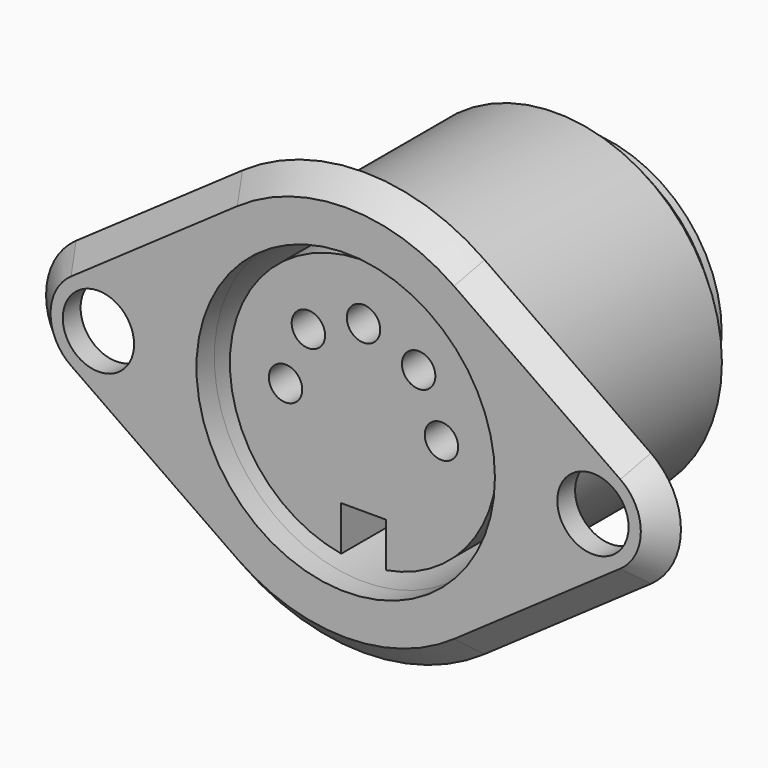
from build123d import *

# Parameters (mm, degrees)
F0_R     = 1.6
F0_R_2   = 7.45
F0_R_3   = 6.7
F1_DEPTH = 1
F2_SIZE  = 0.99999
F0_R_4   = 0.75
F3_DEPTH = 12.1
F4_T     = 0.75
F5_DEPTH = 12.6
F6_DEPTH = 10
F7_SIZE  = 1.3


# Not quite as in the source:
# - a fillet or chamfer is up to 0.001 mm smaller than in the source, because OpenCascade refuses the exact size
# - a shell that OpenCascade refuses in one call is made with other operations: the cavity is built on its own and cut out


with BuildPart() as f1:
    # F0 (on Front) → F1 (new body)
    with BuildSketch(Plane.XZ):
        with BuildLine():
            Line((-5.4346846847, 7.7919318771), (-12.902027027, 2.5836405698))
            ThreePointArc((-12.902027027, 2.5836405698), (-14.25, 0), (-12.902027027, -2.5836405698))
            Line((-12.902027027, -2.5836405698), (-5.4346846847, -7.7919318771))
            ThreePointArc((-5.4346846847, -7.7919318771), (0, -9.5), (5.4346846847, -7.7919318771))
            Line((5.4346846847, -7.7919318771), (12.902027027, -2.5836405698))
            ThreePointArc((12.902027027, -2.5836405698), (14.25, 0), (12.902027027, 2.5836405698))
            Line((12.902027027, 2.5836405698), (5.4346846847, 7.7919318771))
            ThreePointArc((5.4346846847, 7.7919318771), (0, 9.5), (-5.4346846847, 7.7919318771))
        make_face()
        with Locations((-11.1, 0)):
            Circle(F0_R, mode=Mode.SUBTRACT)
        Circle(F0_R_2, mode=Mode.SUBTRACT)
        with Locations((11.1, 0)):
            Circle(F0_R, mode=Mode.SUBTRACT)
        Circle(F0_R_2)
        Circle(F0_R_3, mode=Mode.SUBTRACT)
    extrude(amount=F1_DEPTH)

    # F2 (size 1 in the source; OpenCascade refuses exactly that, so slightly less here)
    f2_edges = [f1.edges().sort_by_distance(p)[0] for p in [
        (-9.168356, -1, 5.187786),
        (0, -1, 9.5),
        (-14.25, -1, 0),
        (-9.168356, -1, -5.187786),
        (0, -1, -9.5),
        (9.168356, -1, -5.187786),
        (14.25, -1, 0),
        (9.168356, -1, 5.187786),
    ]]
    chamfer(f2_edges, length=F2_SIZE)

    # F0 (on Front) → F3 (join)
    with BuildSketch(Plane.XZ):
        Circle(F0_R_2)
        Circle(F0_R_3, mode=Mode.SUBTRACT)
        Circle(F0_R_3)
        with BuildLine():
            ThreePointArc((-1, -5.9160797831), (-3.8729833462, 4.582575695), (6, 0))
            ThreePointArc((6, 0), (4.582575695, -3.8729833462), (1, -5.9160797831))
            Line((1, -5.9160797831), (1, -6.3300160691))
            Line((1, -6.3300160691), (-1, -6.3300160691))
            Line((-1, -6.3300160691), (-1, -5.9160797831))
        make_face(mode=Mode.SUBTRACT)
        with BuildLine():
            ThreePointArc((1, -5.9160797831), (4.582575695, -3.8729833462), (6, 0))
            ThreePointArc((6, 0), (-3.8729833462, 4.582575695), (-1, -5.9160797831))
            Line((-1, -5.9160797831), (-1, -3.9160797831))
            Line((-1, -3.9160797831), (0, -3.9160797831))
            Line((0, -3.9160797831), (1, -3.9160797831))
            Line((1, -3.9160797831), (1, -5.9160797831))
        make_face()
        with Locations((-3.5, 0)):
            Circle(F0_R_4, mode=Mode.SUBTRACT)
        with Locations((-2.4748737342, 2.4748737342)):
            Circle(F0_R_4, mode=Mode.SUBTRACT)
        with Locations((3.5, 0)):
            Circle(F0_R_4, mode=Mode.SUBTRACT)
        with Locations((0, 3.5)):
            Circle(F0_R_4, mode=Mode.SUBTRACT)
        with Locations((2.4748737342, 2.4748737342)):
            Circle(F0_R_4, mode=Mode.SUBTRACT)
        with Locations((-3.5, 0)):
            Circle(F0_R_4)
        with Locations((-2.4748737342, 2.4748737342)):
            Circle(F0_R_4)
        with Locations((0, 3.5)):
            Circle(F0_R_4)
        with Locations((2.4748737342, 2.4748737342)):
            Circle(F0_R_4)
        with Locations((3.5, 0)):
            Circle(F0_R_4)
        with BuildLine():
            Line((-1, -3.9160797831), (-1, -5.9160797831))
            ThreePointArc((-1, -5.9160797831), (0, -6), (1, -5.9160797831))
            Line((1, -5.9160797831), (1, -3.9160797831))
            Line((1, -3.9160797831), (0, -3.9160797831))
            Line((0, -3.9160797831), (-1, -3.9160797831))
        make_face()
        with BuildLine():
            ThreePointArc((1, -5.9160797831), (0, -6), (-1, -5.9160797831))
            Line((-1, -5.9160797831), (-1, -6.3300160691))
            Line((-1, -6.3300160691), (1, -6.3300160691))
            Line((1, -6.3300160691), (1, -5.9160797831))
        make_face()
    extrude(amount=-F3_DEPTH)

    # F4: shell of thickness 0.75, made by hand


with BuildPart() as f4_core1:
    # F4_t2: copy of F1
    add(f1.part)

    # the walls: a layer under each face that stays
    f4_faces = [f4_core1.faces().sort_by_distance(p)[0] for p in [
        (0, -5e-06, 9.5),
        (9.1683558559, -5e-06, 5.1877862235),
        (0, -0.500005, 9.000005),
        (-12.2142857143, 0, -2.7142857143),
        (-9.1683558559, -5e-06, 5.1877862235),
        (14.25, -5e-06, 0),
        (8.8823226802, -0.500005, 4.7776886467),
        (-8.83334, -1, 0),
        (-8.8823226802, -0.500005, 4.7776886467),
        (-14.25, -5e-06, 0),
        (9.1683558559, -5e-06, -5.1877862235),
        (-9.1683558559, -5e-06, -5.1877862235),
        (0, -5e-06, -9.5),
        (-12.7, -0.5, 0),
        (-7.45, 6.05, 0),
        (9.5, -0.5, 0),
        (13.750005, -0.500005, 0),
        (-13.750005, -0.500005, 0),
        (-8.8823226802, -0.500005, -4.7776886467),
        (0, -0.500005, -9.000005),
        (8.8823226802, -0.500005, -4.7776886467),
        (-6.7, -0.5, 0),
        (0, 12.1, 0),
    ]]
    thicken(f4_faces, amount=-F4_T, mode=Mode.SUBTRACT)

    # F4_s3 → F4_t4 (revolve, cut)
    with BuildSketch(Plane.XY):
        Polygon((7.4575, 0.0075), (7.45, -0.75), (6.7, -0.75), (6.7, 0), align=None)
    revolve(axis=Axis((0, 0, 0), (0, -1, 0)), mode=Mode.SUBTRACT)


with BuildPart() as f1_1:
    add(f1.part)

    # what is left inside the walls is the cavity
    f4_cavity = [f4_core1.part.solids().sort_by_distance(p)[0] for p in [
        (-6.6925, 7.566667, 0),
    ]]
    add(f4_cavity, mode=Mode.SUBTRACT)

    # F7
    f7_edges = [f1_1.edges().sort_by_distance(p)[0] for p in [
        (-7.45, 12.1, 0),
    ]]
    chamfer(f7_edges, length=F7_SIZE)


with BuildPart() as f5:
    # F0 (on Front) → F5 (new body)
    with BuildSketch(Plane.XZ):
        with BuildLine():
            ThreePointArc((1, -5.9160797831), (4.582575695, -3.8729833462), (6, 0))
            ThreePointArc((6, 0), (-3.8729833462, 4.582575695), (-1, -5.9160797831))
            Line((-1, -5.9160797831), (-1, -3.9160797831))
            Line((-1, -3.9160797831), (0, -3.9160797831))
            Line((0, -3.9160797831), (1, -3.9160797831))
            Line((1, -3.9160797831), (1, -5.9160797831))
        make_face()
        with Locations((-3.5, 0)):
            Circle(F0_R_4, mode=Mode.SUBTRACT)
        with Locations((-2.4748737342, 2.4748737342)):
            Circle(F0_R_4, mode=Mode.SUBTRACT)
        with Locations((3.5, 0)):
            Circle(F0_R_4, mode=Mode.SUBTRACT)
        with Locations((0, 3.5)):
            Circle(F0_R_4, mode=Mode.SUBTRACT)
        with Locations((2.4748737342, 2.4748737342)):
            Circle(F0_R_4, mode=Mode.SUBTRACT)
        with Locations((-3.5, 0)):
            Circle(F0_R_4)
        with Locations((-2.4748737342, 2.4748737342)):
            Circle(F0_R_4)
        with Locations((0, 3.5)):
            Circle(F0_R_4)
        with Locations((2.4748737342, 2.4748737342)):
            Circle(F0_R_4)
        with Locations((3.5, 0)):
            Circle(F0_R_4)
        with BuildLine():
            Line((-1, -3.9160797831), (-1, -5.9160797831))
            ThreePointArc((-1, -5.9160797831), (0, -6), (1, -5.9160797831))
            Line((1, -5.9160797831), (1, -3.9160797831))
            Line((1, -3.9160797831), (0, -3.9160797831))
            Line((0, -3.9160797831), (-1, -3.9160797831))
        make_face()
    extrude(amount=-F5_DEPTH)

    # F0 (on Front) → F6 (cut)
    with BuildSketch(Plane.XZ):
        with Locations((-3.5, 0)):
            Circle(F0_R_4)
        with BuildLine():
            Line((-1, -3.9160797831), (-1, -5.9160797831))
            ThreePointArc((-1, -5.9160797831), (0, -6), (1, -5.9160797831))
            Line((1, -5.9160797831), (1, -3.9160797831))
            Line((1, -3.9160797831), (0, -3.9160797831))
            Line((0, -3.9160797831), (-1, -3.9160797831))
        make_face()
        with Locations((-2.4748737342, 2.4748737342)):
            Circle(F0_R_4)
        with Locations((0, 3.5)):
            Circle(F0_R_4)
        with Locations((2.4748737342, 2.4748737342)):
            Circle(F0_R_4)
        with Locations((3.5, 0)):
            Circle(F0_R_4)
    extrude(amount=-F6_DEPTH, mode=Mode.SUBTRACT)


solid = Compound([f1_1.part, f5.part])
